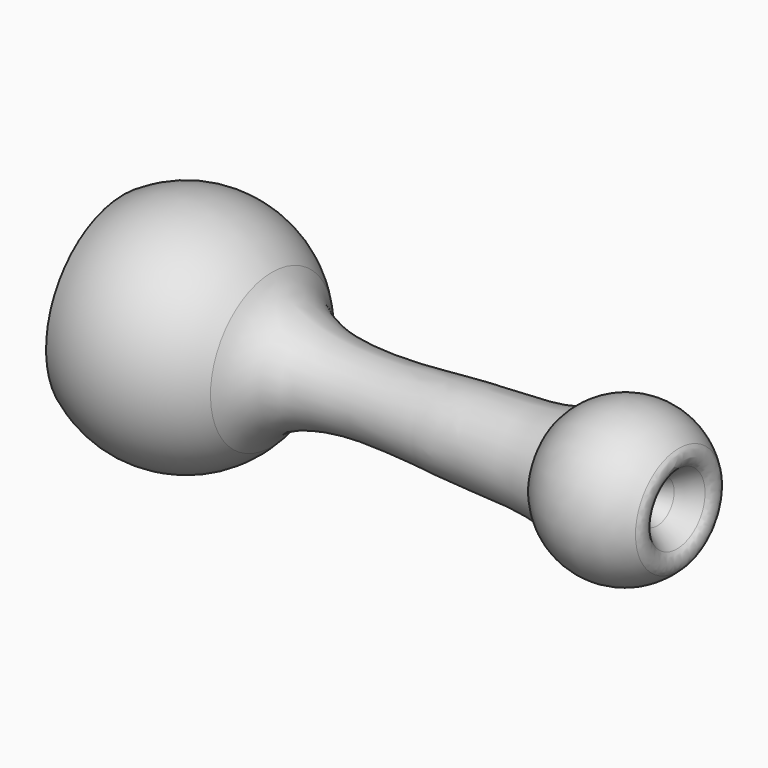
from build123d import *

# Parameters (mm, degrees)
F2_R = 2
F3_R = 5


with BuildPart() as f1:
    # F0 (on Front) → F1 (revolve)
    with BuildSketch(Plane.XZ):
        with BuildLine():
            ThreePointArc((-7.0685046336, 10.3095219212), (4.6853520259, 11.5886788028), (12.2474487139, 2.5))
            Line((12.2474487139, 2.5), (74.2474487139, 2.5))
            Line((74.2474487139, 2.5), (80.4566636234, 6.848955093))
            ThreePointArc((80.4566636234, 6.848955093), (71.1861926887, 12.2493617225), (61.3018820008, 8.0772608919))
            add(Edge.make_bspline(
                [(13.7809895682, 12.3177978136), (18.9431640709, 3.8047084098), (45.8510372203, 7.5452258089), (55.5286329868, 6.7225269235), (61.3018820008, 8.0772608919)],
                knots=[0, 0, 0, 0, 0.5718996335, 1, 1, 1, 1], degree=3))
            ThreePointArc((13.7809895682, 12.3177978136), (2.4835532955, 18.3159979112), (-10.003236638, 15.5428141988))
            Line((-10.003236638, 15.5428141988), (-7.0685046336, 10.3095219212))
        make_face()
    revolve(axis=Axis((35, 0, 0), (1, 0, 0)))

    # F2
    f2_edges = [f1.edges().sort_by_distance(p)[0] for p in [
        (80.456664, 0, -6.848955),
        (-7.068505, 0, -10.309522),
        (12.247449, 0, -2.5),
    ]]
    fillet(f2_edges, radius=F2_R)

    # F3
    f3_edges = [f1.edges().sort_by_distance(p)[0] for p in [
        (74.247449, 0, -2.5),
    ]]
    fillet(f3_edges, radius=F3_R)


solid = f1.part
